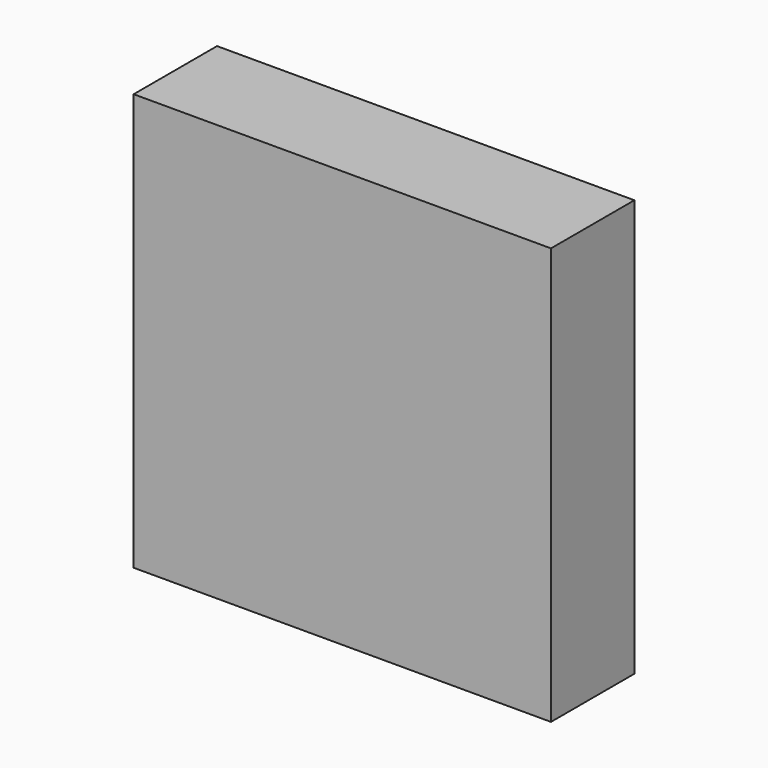
from build123d import *

# Parameters (mm, degrees)
F1_E0_BOTTOM_W = 100.1032665372
F1_E0_BOTTOM_H = 100
F2_DEPTH       = 25


with BuildPart() as f2:
    # F1_E0_bottom (on explicit) → F2 (new body)
    with BuildSketch(Plane(origin=(50.0516332686, 50.1900725067, 0), x_dir=(-1, 0, 0), z_dir=(0, 1, 0))):
        with Locations((50.0516332686, 50)):
            Rectangle(F1_E0_BOTTOM_W, F1_E0_BOTTOM_H)
    extrude(amount=F2_DEPTH)


solid = f2.part
